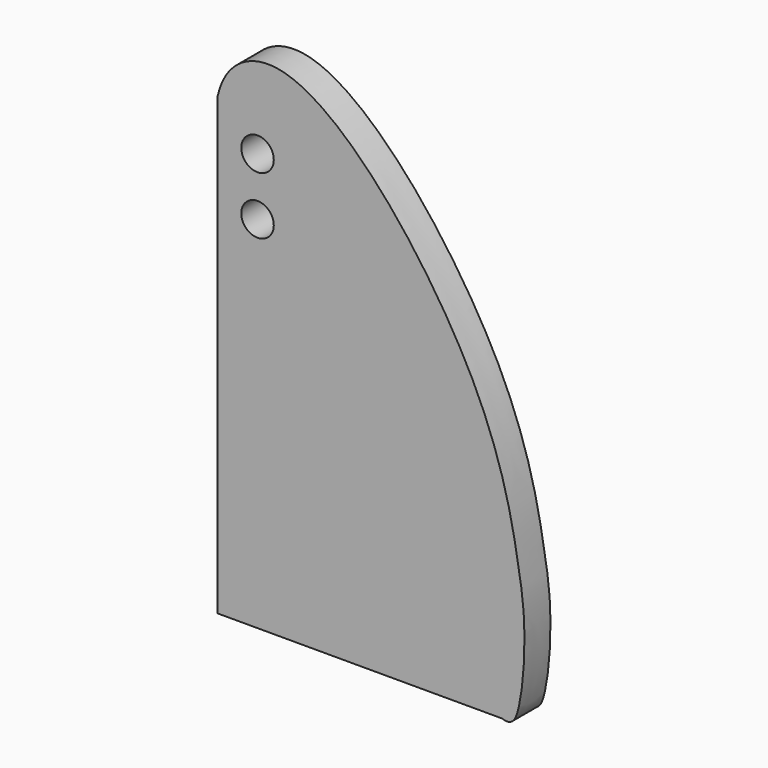
from build123d import *

# Parameters (mm, degrees)
F0_R     = 6.35
F1_DEPTH = 12.7


with BuildPart() as f1:
    # F0 (on Front) → F1 (new body)
    with BuildSketch(Plane.XZ):
        with BuildLine():
            Line((-62.4917310791, 62.3387722267), (-62.4917310791, -98.4021690574))
            Line((-62.4917310791, -98.4021690574), (48.7352559237, -98.4021690574))
            add(Edge.make_bspline(
                [(48.7352559237, -98.4021690574), (29.3297900082, -91.6985332362), (-53.7117630872, 10.9735691095), (-62.4917310791, 62.3387722267)],
                knots=[0.7299039405, 0.7299039405, 0.7299039405, 0.7299039405, 1, 1, 1, 1], degree=3))
        make_face()
        with BuildLine():
            add(Edge.make_bspline(
                [(48.7352559237, -98.4021690574), (29.3297900082, -91.6985332362), (-53.7117630872, 10.9735691095), (-62.4917310791, 62.3387722267)],
                knots=[0.7299039405, 0.7299039405, 0.7299039405, 0.7299039405, 1, 1, 1, 1], degree=3))
            add(Edge.make_bspline(
                [(-62.4917310791, 79.3978309426), (-59.8076427315, 91.8791864682), (-30.3583811457, 112.2582538654), (43.3116486469, 19.975292811), (54.796151396, -40.6196685771), (58.3164600027, -64.1777234903), (56.4358345174, -92.3455133169), (52.6766606255, -99.7637308905), (48.7352559237, -98.4021690574)],
                knots=[0.03442933, 0.03442933, 0.03442933, 0.03442933, 0.1239997664, 0.3250967159, 0.4796932186, 0.573227326, 0.6750452793, 0.7299039405, 0.7299039405, 0.7299039405, 0.7299039405], degree=3))
            Line((-62.4917310791, 79.3978309426), (-62.4917310791, 62.3387722267))
        make_face()
        with Locations((-46.8575544655, 42.2490648925)):
            Circle(F0_R, mode=Mode.SUBTRACT)
        with Locations((-46.8575544655, 64.7881403565)):
            Circle(F0_R, mode=Mode.SUBTRACT)
    extrude(amount=F1_DEPTH)


solid = f1.part
